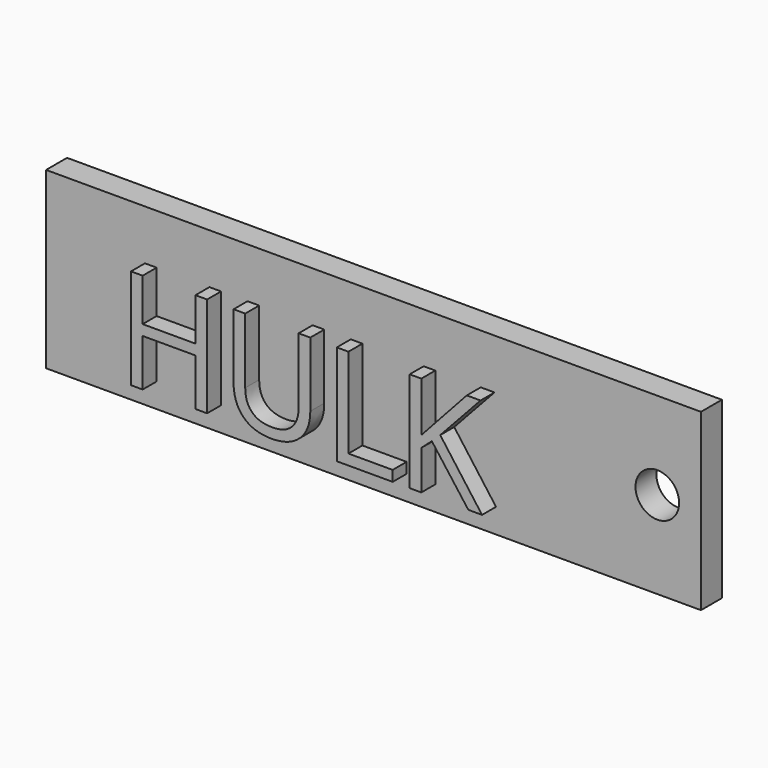
from build123d import *

# Parameters (mm, degrees)
F0_W         = 75
F0_H         = 20
F0_R         = 2.5
F1_DEPTH     = 3
F2_TEXT_SIZE = 16.0783367594
F3_DEPTH     = 2


# Not quite as in the source:
# - Text() gives the source's letters only with a copy of the font that has no kerning and outlines rounded to 1/6400 em; it was checked with that copy


with BuildPart() as f1:
    # F0 (on Front) → F1 (new body)
    with BuildSketch(Plane.XZ):
        with Locations((37.5, -10)):
            Rectangle(F0_W, F0_H)
        with Locations((70, -10)):
            Circle(F0_R, mode=Mode.SUBTRACT)
    extrude(amount=-F1_DEPTH)

    # F2 (on face) → F3 (join)
    with BuildSketch(Plane.XZ):
        with Locations((9.7485492006, -17.2122828662)):
            Text('HULK', F2_TEXT_SIZE, font='Open Sans', text_align=(TextAlign.LEFT, TextAlign.BOTTOM))
    extrude(amount=F3_DEPTH)


solid = f1.part
